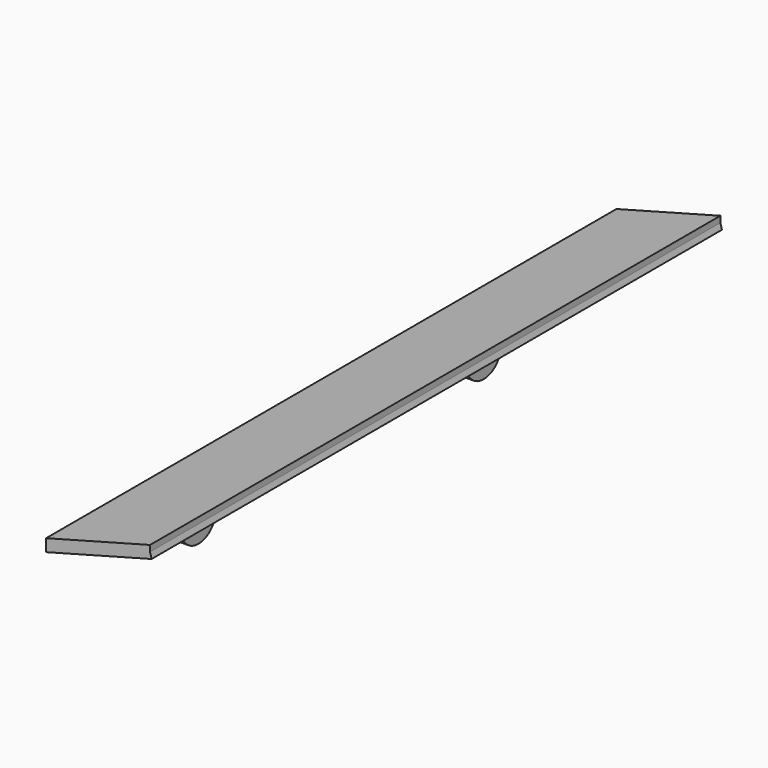
from build123d import *

# Parameters (mm, degrees)
F2_DEPTH  = 120
F3_W      = 36.2346663144
F3_H      = 240
F3_W_2    = 2.2
F3_H_2    = 235.6
F4_DEPTH  = 2
F5_R      = 2
F7_DEPTH  = 240
F8_W      = 15
F8_H      = 4.1411047216
F8_H_2    = 20.8588952784
F8_R      = 2
F9_DEPTH  = 3.3
F10_R     = 7.49999
F11_W     = 2.2
F11_H     = 25.02
F12_DEPTH = 2
F13_R     = 5
F14_R     = 7


# Not quite as in the source:
# - a fillet or chamfer is up to 0.001 mm smaller than in the source, because OpenCascade refuses the exact size
# - a feature names something its author has since deleted; it is built from what else it names


with BuildPart() as f2:
    # F1 (on Front) → F2 (new body, symmetric)
    with BuildSketch(Plane.XZ):
        Polygon((35, 11.4487740959), (0, 2.0705523608), (0, 0), (35, 9.3782217351), align=None)
    extrude(amount=F2_DEPTH, both=True)

    # F3 (on face) → F4 (join)
    with BuildSketch(Plane(origin=(0, 0, 0), x_dir=(0.9659258263, 0, 0.2588190451), z_dir=(0.2588190451, 0, -0.9659258263))):
        with Locations((18.1173331572, 0)):
            Rectangle(F3_W, F3_H)
        Polygon((2.2, -117.8), (2.2, 117.8), (6.4057777191, 117.8), (8.6057777191, 117.8), (17.0173331572, 117.8), (19.2173331572, 117.8), (27.6288885953, 117.8), (29.8288885953, 117.8), (34.0346663144, 117.8), (34.0346663144, -117.8), (29.8288885953, -117.8), (27.6288885953, -117.8), (19.2173331572, -117.8), (17.0173331572, -117.8), (8.6057777191, -117.8), (6.4057777191, -117.8), align=None, mode=Mode.SUBTRACT)
        with Locations((28.7288885953, 0)):
            Rectangle(F3_W_2, F3_H_2)
        with Locations((18.1173331572, 0)):
            Rectangle(F3_W_2, F3_H_2)
        with Locations((7.5057777191, 0)):
            Rectangle(F3_W_2, F3_H_2)
    extrude(amount=F4_DEPTH)

    # F5
    f5_edges = [f2.edges().sort_by_distance(p)[0] for p in [
        (33.133782, -117.8, 7.842894),
        (26.946276, -117.8, 6.184957),
        (16.696301, -117.8, 3.438484),
        (6.446325, -117.8, 0.692011),
        (29.071313, -117.8, 6.754359),
        (18.821337, -117.8, 4.007886),
        (8.571362, -117.8, 1.261413),
        (2.383856, -117.8, -0.396524),
        (2.383856, 117.8, -0.396524),
        (8.571362, 117.8, 1.261413),
        (18.821337, 117.8, 4.007886),
        (29.071313, 117.8, 6.754359),
        (33.133782, 117.8, 7.842894),
        (16.696301, 117.8, 3.438484),
        (6.446325, 117.8, 0.692011),
        (26.946276, 117.8, 6.184957),
    ]]
    fillet(f5_edges, radius=F5_R)

    # F6 (on face) → F7 (join, through all)
    with BuildSketch(Plane.XZ.offset(120)):
        Polygon((0, -2.0705523608), (0.5176380902, -1.9318516526), (0, 0), align=None)
    extrude(amount=-F7_DEPTH)

    # F8 (on face) → F9 (join)
    with BuildSketch(Plane(origin=(0, 0, 0), x_dir=(0, -1, 0), z_dir=(-1, 0, 0))):
        with Locations((-60, 0)):
            Rectangle(F8_W, F8_H)
        with Locations((-60, -12.5)):
            Rectangle(F8_W, F8_H_2)
        with Locations((-60, -15.9294476392)):
            Circle(F8_R, mode=Mode.SUBTRACT)
        with Locations((60, 0)):
            Rectangle(F8_W, F8_H)
        with Locations((60, -12.5)):
            Rectangle(F8_W, F8_H_2)
        with Locations((60, -15.9294476392)):
            Circle(F8_R, mode=Mode.SUBTRACT)
    extrude(amount=-F9_DEPTH)

    # F10 (radius 7.5 in the source; OpenCascade refuses exactly that, so slightly less here)
    f10_edges = [f2.edges().sort_by_distance(p)[0] for p in [
        (1.65, 67.5, -22.929448),
        (1.65, 52.5, -22.929448),
        (1.65, -52.5, -22.929448),
        (1.65, -67.5, -22.929448),
    ]]
    fillet(f10_edges, radius=F10_R)

    # F11 (on face) → F12 (join, through all)
    with BuildSketch(Plane(origin=(0.5176380902, 0, -1.9318516526), x_dir=(0.9659258263, 0, 0.2588190451), z_dir=(0.2588190451, 0, -0.9659258263))):
        Polygon((6.4057777191, -47.49), (2.2, -47.49), (2.2, -52.5), (2.2, -67.5), (2.2, -72.51), (6.4057777191, -72.51), align=None)
        with Locations((7.5057777191, -60)):
            Rectangle(F11_W, F11_H)
        Polygon((2.2, 52.5), (2.2, 47.49), (6.4057777191, 47.49), (6.4057777191, 72.51), (2.2, 72.51), (2.2, 67.5), align=None)
        with Locations((7.5057777191, 60)):
            Rectangle(F11_W, F11_H)
    extrude(amount=-F12_DEPTH)

    # F13
    f13_edges = [f2.edges().sort_by_distance(p)[0] for p in [
        (1.65, -52.5, -1.628436),
        (1.65, -67.5, -1.628436),
        (1.65, 52.5, -1.628436),
        (1.65, 67.5, -1.628436),
    ]]
    fillet(f13_edges, radius=F13_R)

    # F14
    f14_edges = [f2.edges().sort_by_distance(p)[0] for p in [
        (3.3, 60, -1.18632),
        (3.3, -60, -1.18632),
    ]]
    fillet(f14_edges, radius=F14_R)


solid = f2.part
